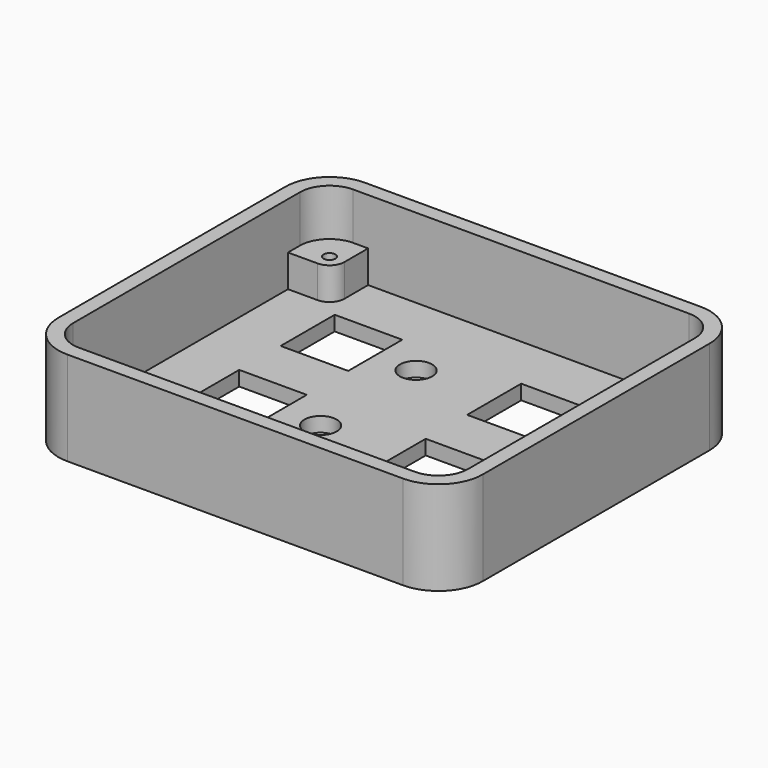
from build123d import *

# Parameters (mm, degrees)
F1_DEPTH         = 16
F2_T             = -2.5
F3_R             = 1
F4_DEPTH         = 5.5
F4_COPIES2_COUNT = 2
F5_W             = 11.5
F5_H             = 11.5
F5_R             = 2.75
F6_DEPTH         = 2.501


# Not quite as in the source:
# - a pattern or mirror of a feature is missing from the dataset's text; its kind, count and spacing are read off the source's solid


with BuildPart() as f1:
    # F0 (on Top) → F1 (new body)
    with BuildSketch(Plane.XY):
        with BuildLine():
            ThreePointArc((36.12, 24.13), (33.9115851301, 29.4615851301), (28.58, 31.67))
            Line((28.58, 31.67), (-28.58, 31.67))
            ThreePointArc((-28.58, 31.67), (-33.9115851301, 29.4615851301), (-36.12, 24.13))
            Line((-36.12, 24.13), (-36.12, -24.13))
            ThreePointArc((-36.12, -24.13), (-33.9115851301, -29.4615851301), (-28.58, -31.67))
            Line((-28.58, -31.67), (28.58, -31.67))
            ThreePointArc((28.58, -31.67), (33.9115851301, -29.4615851301), (36.12, -24.13))
            Line((36.12, -24.13), (36.12, 24.13))
        make_face()
    extrude(amount=F1_DEPTH)

    # F2
    f2_openings = [f1.faces().sort_by_distance(p)[0] for p in [
        (0, 0, 16),
    ]]
    offset(amount=F2_T, openings=f2_openings)

    # F3 (on face) → F4 (join)
    with BuildSketch(Plane.XY.offset(2.5)):
        with BuildLine():
            Line((-26.04, 24.13), (-26.04, 29.17))
            Line((-26.04, 29.17), (-28.58, 29.17))
            ThreePointArc((-28.58, 29.17), (-32.1438181772, 27.6938181772), (-33.62, 24.13))
            Line((-33.62, 24.13), (-33.62, 21.59))
            Line((-33.62, 21.59), (-28.58, 21.59))
            ThreePointArc((-28.58, 21.59), (-26.7839487758, 22.3339487758), (-26.04, 24.13))
        make_face()
        with Locations((-28.58, 24.13)):
            Circle(F3_R, mode=Mode.SUBTRACT)
    f4 = extrude(amount=F4_DEPTH)

    # F4_copies: F4 across plane
    add(f4.mirror(Plane(origin=(0, 0, 0), x_dir=(0, 0, 1), z_dir=(1, 0, 0))))

    # F4_copies1: F4 across plane
    add(f4.mirror(Plane(origin=(0, 0, 0), x_dir=(0, 0, -1), z_dir=(0, -1, 0))))

    # F4_copies2: F4 ×2 about axis
    f4_copies2_axis = Axis((0, 0, 0), (0, 0, 1))
    for i in range(1, F4_COPIES2_COUNT):
        add(f4.rotate(f4_copies2_axis, i * 360 / F4_COPIES2_COUNT))

    # F5 (on face) → F6 (cut, through all)
    with BuildSketch(Plane.XY.offset(2.5)):
        with Locations((-18.42, 13.97)):
            Rectangle(F5_W, F5_H)
        with Locations((-5.72, 13.97)):
            Circle(F5_R)
        with Locations((-18.42, -6.35)):
            Rectangle(F5_W, F5_H)
        with Locations((-5.72, -6.35)):
            Circle(F5_R)
        with Locations((13.33, 13.97)):
            Rectangle(F5_W, F5_H)
        with Locations((26.03, 13.97)):
            Circle(F5_R)
        with Locations((13.33, -6.35)):
            Rectangle(F5_W, F5_H)
        with Locations((26.03, -6.35)):
            Circle(F5_R)
    extrude(amount=-F6_DEPTH, mode=Mode.SUBTRACT)


solid = f1.part
